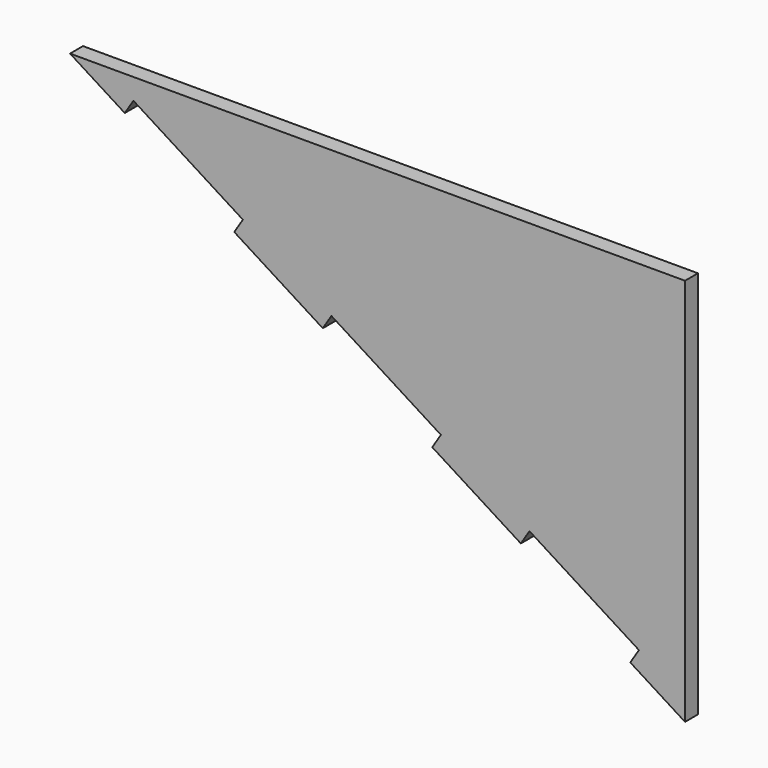
from build123d import *

# Parameters (mm, degrees)
F1_DEPTH = 3.175


# Not quite as in the source:
# - a feature names something its author has since deleted; it is built from what else it names


with BuildPart() as f1:
    # F0 (on Front) → F1 (new body)
    with BuildSketch(Plane.XZ):
        Polygon((57.7196001889, 0), (-62.9303998111, 0), (-52.1926907426, -6.7817109906), (-50.4972629949, -4.0972837235), (-29.0218448579, -17.6607057048), (-30.7172726056, -20.3451329719), (-13.3431088796, -31.3182890094), (-11.6476811319, -28.6338617422), (-0.9099720634, -35.4155727329), (9.8277370051, -42.1972837235), (8.1323092574, -44.8817109906), (25.5064729834, -55.8548670281), (27.2019007311, -53.170439761), (48.6773188681, -66.7338617422), (46.9818911204, -69.4182890094), (57.7196001889, -76.2), align=None)
    extrude(amount=F1_DEPTH)


solid = f1.part
